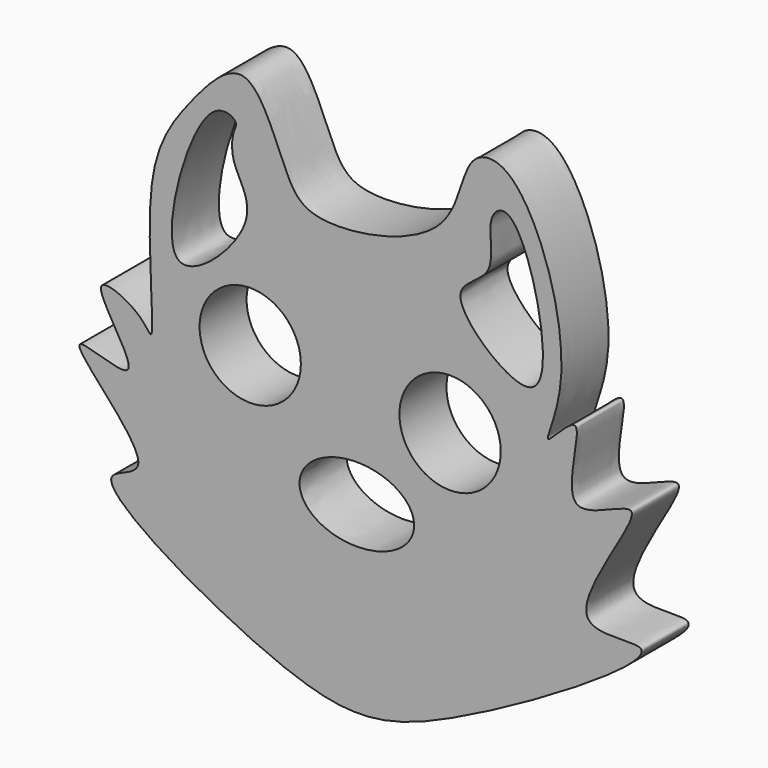
from build123d import *

# Parameters (mm, degrees)
F0_R     = 10.9404020296
F3_DEPTH = 12.7


# Not quite as in the source:
# - a feature of the source that left no trace in its solid (it failed there, or was rolled back) is left out


with BuildPart() as f3:
    # F0 (on Front) → F3 (new body)
    with BuildSketch(Plane.XZ):
        with BuildLine():
            add(Edge.make_bspline(
                [(-44.3963385475, 11.0176274683), (-43.5956904498, 12.2226852091), (-47.0807262057, 42.1894243845), (-37.7066996439, 56.2735408751), (-23.2144452715, 72.944861215), (-15.6807960515, 50.9371724364), (-9.8001740811, 42.1994319683), (22.3420627671, 47.9778289448), (22.4809617418, 68.1653128947), (36.5388778271, 69.4906114026), (48.7162678599, 32.960535246), (37.9488306631, 14.1200838192), (51.4039847015, 30.2555110719), (41.0440196393, 0.404790861), (69.9654721483, 20.5033650724), (38.6730995153, -18.5240711957), (77.2629587468, -8.872144765), (14.9736101781, -46.5560659508), (-9.7688291438, -49.4684506631), (-64.2877801424, -17.694996921), (-38.806925616, -16.7515375496), (-70.8278372437, 10.869064196), (-41.2267882542, -3.6326312985), (-61.6487998945, 21.1149363264), (-46.3888953433, 14.6691576653), (-44.6999119452, 10.5607182794), (-44.3963385475, 11.0176274683)],
                knots=[0, 0, 0, 0, 0.0524994782, 0.0983817078, 0.1363256126, 0.1774839098, 0.2094888309, 0.261404062, 0.3015248535, 0.3294078242, 0.3908119696, 0.4250518051, 0.4516067603, 0.4899319062, 0.5246367957, 0.5746304686, 0.608902938, 0.6782538291, 0.7388010908, 0.8054997312, 0.8326568059, 0.8799471359, 0.912297769, 0.9509931096, 0.9800943198, 1, 1, 1, 1], degree=3))
        make_face()
        with BuildLine():
            add(Edge.make_bspline(
                [(-12.3756472021, -6.9073382765), (-12.3756472021, -14.9419499698), (0, -14.9419499698)],
                knots=[0, 0, 0, 1.5707963268, 1.5707963268, 1.5707963268], degree=2, weights=[1, 0.7071067812, 1]))
            add(Edge.make_bspline(
                [(0, -14.9419499698), (29.8774553185, -14.9419499698), (8.7509040582, -1.226009864), (-12.3756472021, 12.4899302418), (-12.3756472021, -6.9073382765)],
                knots=[1.5707963268, 1.5707963268, 1.5707963268, 3.926990817, 3.926990817, 6.2831853072, 6.2831853072, 6.2831853072], degree=2, weights=[1, 0.3826834324, 1, 0.3826834324, 1]))
        make_face(mode=Mode.SUBTRACT)
        with BuildLine():
            add(Edge.make_bspline(
                [(-24.0906851895, 38.8852398546), (-22.6271256395, 43.4233212193), (-27.5918384294, 48.6350615893), (-26.8110432735, 55.444402584), (-25.3707126452, 57.4975608293), (-34.3600765379, 62.120877975), (-47.4089262083, 13.1575254952), (-26.0089752136, 32.9371687903), (-24.0906851895, 38.8852398546)],
                knots=[0, 0, 0, 0, 0.1716125209, 0.2995049816, 0.3683361725, 0.483504911, 0.7750671731, 1, 1, 1, 1], degree=3))
        make_face(mode=Mode.SUBTRACT)
        with Locations((-23.024648428, 15.8289410174)):
            Circle(F0_R, mode=Mode.SUBTRACT)
        with Locations((20.1464034617, 13.2390642539)):
            Circle(F0_R, mode=Mode.SUBTRACT)
        with BuildLine():
            add(Edge.make_bspline(
                [(22.3892752205, 39.8891382027), (22.303190844, 42.8729025083), (31.2940107754, 45.2060403839), (27.3717334541, 56.7054467821), (33.922773798, 61.9434163354), (41.0567706657, 41.0385457672), (40.1087481888, 20.281270185), (22.514915746, 35.5343210966), (22.3892752205, 39.8891382027)],
                knots=[0, 0, 0, 0, 0.1446254066, 0.2987807385, 0.3947037119, 0.6123248029, 0.788918584, 1, 1, 1, 1], degree=3))
        make_face(mode=Mode.SUBTRACT)
    extrude(amount=F3_DEPTH)


solid = f3.part
